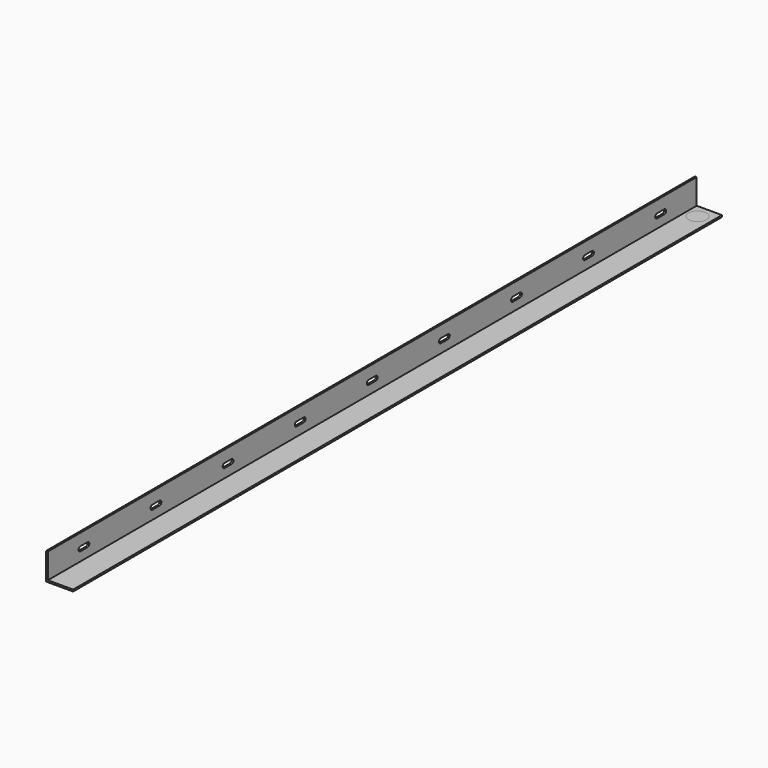
from build123d import *

# Parameters (mm, degrees)
F1_DEPTH = 400
F3_DEPTH = 2
F4_DEPTH = 900
F5_DEPTH = 2
F6_R     = 10
F7_DEPTH = 2


with BuildPart() as f1:
    # F0 (on Front) → F1 (new body)
    with BuildSketch(Plane.XZ):
        Polygon((-6.9707836596, 25.3386970109), (-8.9707836596, 25.3386970109), (-8.9707836596, -4.6613029891), (21.0292163404, -4.6613029891), (21.0292163404, -2.6613029891), (-6.9707836596, -2.6613029891), align=None)
    extrude(amount=F1_DEPTH)

    # F2 (on face) → F3 (cut)
    with BuildSketch(Plane.YZ.offset(-6.9707836596)):
        with BuildLine():
            ThreePointArc((-352.5, 9.7042359412), (-351.767766953, 11.4720028941), (-350, 12.2042359412))
            Line((-350, 12.2042359412), (-355, 12.2042359412))
            ThreePointArc((-355, 12.2042359412), (-357.5, 9.7042359412), (-355, 7.2042359412))
            Line((-355, 7.2042359412), (-350, 7.2042359412))
            ThreePointArc((-350, 7.2042359412), (-351.767766953, 7.9364689882), (-352.5, 9.7042359412))
        make_face()
        with BuildLine():
            Line((-347.5, 9.7042359412), (-350, 9.7042359412))
            Line((-350, 9.7042359412), (-350, 7.2042359412))
            ThreePointArc((-350, 7.2042359412), (-348.232233047, 7.9364689882), (-347.5, 9.7042359412))
        make_face()
        with BuildLine():
            Line((-350, 7.2042359412), (-350, 9.7042359412))
            Line((-350, 9.7042359412), (-352.5, 9.7042359412))
            ThreePointArc((-352.5, 9.7042359412), (-351.767766953, 7.9364689882), (-350, 7.2042359412))
        make_face()
        with BuildLine():
            ThreePointArc((-347.5, 9.7042359412), (-348.232233047, 11.4720028941), (-350, 12.2042359412))
            Line((-350, 12.2042359412), (-350, 9.7042359412))
            Line((-350, 9.7042359412), (-347.5, 9.7042359412))
        make_face()
        with BuildLine():
            Line((-345, 12.2042359412), (-350, 12.2042359412))
            ThreePointArc((-350, 12.2042359412), (-348.232233047, 11.4720028941), (-347.5, 9.7042359412))
            ThreePointArc((-347.5, 9.7042359412), (-348.232233047, 7.9364689882), (-350, 7.2042359412))
            Line((-350, 7.2042359412), (-345, 7.2042359412))
            ThreePointArc((-345, 7.2042359412), (-342.5, 9.7042359412), (-345, 12.2042359412))
        make_face()
        with BuildLine():
            Line((-350, 9.7042359412), (-350, 12.2042359412))
            ThreePointArc((-350, 12.2042359412), (-351.767766953, 11.4720028941), (-352.5, 9.7042359412))
            Line((-352.5, 9.7042359412), (-350, 9.7042359412))
        make_face()
        with BuildLine():
            Line((-255, 7.2042359412), (-250, 7.2042359412))
            Line((-250, 7.2042359412), (-245, 7.2042359412))
            ThreePointArc((-245, 7.2042359412), (-242.5, 9.7042359412), (-245, 12.2042359412))
            Line((-245, 12.2042359412), (-250, 12.2042359412))
            Line((-250, 12.2042359412), (-255, 12.2042359412))
            ThreePointArc((-255, 12.2042359412), (-257.5, 9.7042359412), (-255, 7.2042359412))
        make_face()
        with BuildLine():
            Line((-155, 7.2042359412), (-150, 7.2042359412))
            Line((-150, 7.2042359412), (-145, 7.2042359412))
            ThreePointArc((-145, 7.2042359412), (-142.5, 9.7042359412), (-145, 12.2042359412))
            Line((-145, 12.2042359412), (-150, 12.2042359412))
            Line((-150, 12.2042359412), (-155, 12.2042359412))
            ThreePointArc((-155, 12.2042359412), (-157.5, 9.7042359412), (-155, 7.2042359412))
        make_face()
        with BuildLine():
            Line((-55, 7.2042359412), (-50, 7.2042359412))
            Line((-50, 7.2042359412), (-45, 7.2042359412))
            ThreePointArc((-45, 7.2042359412), (-42.5, 9.7042359412), (-45, 12.2042359412))
            Line((-45, 12.2042359412), (-50, 12.2042359412))
            Line((-50, 12.2042359412), (-55, 12.2042359412))
            ThreePointArc((-55, 12.2042359412), (-57.5, 9.7042359412), (-55, 7.2042359412))
        make_face()
    extrude(amount=-F3_DEPTH, mode=Mode.SUBTRACT)


with BuildPart() as f4:
    # F0 (on Front) → F4 (new body)
    with BuildSketch(Plane.XZ):
        Polygon((-6.9707836596, 25.3386970109), (-8.9707836596, 25.3386970109), (-8.9707836596, -4.6613029891), (21.0292163404, -4.6613029891), (21.0292163404, -2.6613029891), (-6.9707836596, -2.6613029891), align=None)
    extrude(amount=F4_DEPTH)

    # F2 (on face) → F5 (cut)
    with BuildSketch(Plane.YZ.offset(-6.9707836596)):
        with BuildLine():
            ThreePointArc((-347.5, 9.7042359412), (-348.232233047, 11.4720028941), (-350, 12.2042359412))
            Line((-350, 12.2042359412), (-350, 9.7042359412))
            Line((-350, 9.7042359412), (-347.5, 9.7042359412))
        make_face()
        with BuildLine():
            Line((-345, 12.2042359412), (-350, 12.2042359412))
            ThreePointArc((-350, 12.2042359412), (-348.232233047, 11.4720028941), (-347.5, 9.7042359412))
            ThreePointArc((-347.5, 9.7042359412), (-348.232233047, 7.9364689882), (-350, 7.2042359412))
            Line((-350, 7.2042359412), (-345, 7.2042359412))
            ThreePointArc((-345, 7.2042359412), (-342.5, 9.7042359412), (-345, 12.2042359412))
        make_face()
        with BuildLine():
            ThreePointArc((-352.5, 9.7042359412), (-351.767766953, 11.4720028941), (-350, 12.2042359412))
            Line((-350, 12.2042359412), (-355, 12.2042359412))
            ThreePointArc((-355, 12.2042359412), (-357.5, 9.7042359412), (-355, 7.2042359412))
            Line((-355, 7.2042359412), (-350, 7.2042359412))
            ThreePointArc((-350, 7.2042359412), (-351.767766953, 7.9364689882), (-352.5, 9.7042359412))
        make_face()
        with BuildLine():
            Line((-350, 9.7042359412), (-350, 12.2042359412))
            ThreePointArc((-350, 12.2042359412), (-351.767766953, 11.4720028941), (-352.5, 9.7042359412))
            Line((-352.5, 9.7042359412), (-350, 9.7042359412))
        make_face()
        with BuildLine():
            Line((-347.5, 9.7042359412), (-350, 9.7042359412))
            Line((-350, 9.7042359412), (-350, 7.2042359412))
            ThreePointArc((-350, 7.2042359412), (-348.232233047, 7.9364689882), (-347.5, 9.7042359412))
        make_face()
        with BuildLine():
            Line((-350, 7.2042359412), (-350, 9.7042359412))
            Line((-350, 9.7042359412), (-352.5, 9.7042359412))
            ThreePointArc((-352.5, 9.7042359412), (-351.767766953, 7.9364689882), (-350, 7.2042359412))
        make_face()
        with BuildLine():
            Line((-255, 7.2042359412), (-250, 7.2042359412))
            Line((-250, 7.2042359412), (-245, 7.2042359412))
            ThreePointArc((-245, 7.2042359412), (-242.5, 9.7042359412), (-245, 12.2042359412))
            Line((-245, 12.2042359412), (-250, 12.2042359412))
            Line((-250, 12.2042359412), (-255, 12.2042359412))
            ThreePointArc((-255, 12.2042359412), (-257.5, 9.7042359412), (-255, 7.2042359412))
        make_face()
        with BuildLine():
            Line((-155, 7.2042359412), (-150, 7.2042359412))
            Line((-150, 7.2042359412), (-145, 7.2042359412))
            ThreePointArc((-145, 7.2042359412), (-142.5, 9.7042359412), (-145, 12.2042359412))
            Line((-145, 12.2042359412), (-150, 12.2042359412))
            Line((-150, 12.2042359412), (-155, 12.2042359412))
            ThreePointArc((-155, 12.2042359412), (-157.5, 9.7042359412), (-155, 7.2042359412))
        make_face()
        with BuildLine():
            Line((-55, 7.2042359412), (-50, 7.2042359412))
            Line((-50, 7.2042359412), (-45, 7.2042359412))
            ThreePointArc((-45, 7.2042359412), (-42.5, 9.7042359412), (-45, 12.2042359412))
            Line((-45, 12.2042359412), (-50, 12.2042359412))
            Line((-50, 12.2042359412), (-55, 12.2042359412))
            ThreePointArc((-55, 12.2042359412), (-57.5, 9.7042359412), (-55, 7.2042359412))
        make_face()
        with BuildLine():
            ThreePointArc((-445, 7.2042359412), (-442.5, 9.7042359412), (-445, 12.2042359412))
            Line((-445, 12.2042359412), (-450, 12.2042359412))
            Line((-450, 12.2042359412), (-455, 12.2042359412))
            ThreePointArc((-455, 12.2042359412), (-457.5, 9.7042359412), (-455, 7.2042359412))
            Line((-455, 7.2042359412), (-450, 7.2042359412))
            Line((-450, 7.2042359412), (-445, 7.2042359412))
        make_face()
        with BuildLine():
            ThreePointArc((-545, 7.2042359412), (-542.5, 9.7042359412), (-545, 12.2042359412))
            Line((-545, 12.2042359412), (-550, 12.2042359412))
            Line((-550, 12.2042359412), (-555, 12.2042359412))
            ThreePointArc((-555, 12.2042359412), (-557.5, 9.7042359412), (-555, 7.2042359412))
            Line((-555, 7.2042359412), (-550, 7.2042359412))
            Line((-550, 7.2042359412), (-545, 7.2042359412))
        make_face()
        with BuildLine():
            ThreePointArc((-645, 7.2042359412), (-642.5, 9.7042359412), (-645, 12.2042359412))
            Line((-645, 12.2042359412), (-650, 12.2042359412))
            Line((-650, 12.2042359412), (-655, 12.2042359412))
            ThreePointArc((-655, 12.2042359412), (-657.5, 9.7042359412), (-655, 7.2042359412))
            Line((-655, 7.2042359412), (-650, 7.2042359412))
            Line((-650, 7.2042359412), (-645, 7.2042359412))
        make_face()
        with BuildLine():
            ThreePointArc((-745, 7.2042359412), (-742.5, 9.7042359412), (-745, 12.2042359412))
            Line((-745, 12.2042359412), (-750, 12.2042359412))
            Line((-750, 12.2042359412), (-755, 12.2042359412))
            ThreePointArc((-755, 12.2042359412), (-757.5, 9.7042359412), (-755, 7.2042359412))
            Line((-755, 7.2042359412), (-750, 7.2042359412))
            Line((-750, 7.2042359412), (-745, 7.2042359412))
        make_face()
        with BuildLine():
            ThreePointArc((-845, 7.2042359412), (-842.5, 9.7042359412), (-845, 12.2042359412))
            Line((-845, 12.2042359412), (-850, 12.2042359412))
            Line((-850, 12.2042359412), (-855, 12.2042359412))
            ThreePointArc((-855, 12.2042359412), (-857.5, 9.7042359412), (-855, 7.2042359412))
            Line((-855, 7.2042359412), (-850, 7.2042359412))
            Line((-850, 7.2042359412), (-845, 7.2042359412))
        make_face()
    extrude(amount=-F5_DEPTH, mode=Mode.SUBTRACT)

    # F6 (on face) → F7 (cut)
    with BuildSketch(Plane(origin=(0, 0, -4.6613029891), x_dir=(1, 0, 0), z_dir=(0, 0, -1))):
        with Locations((6.0292163404, 15)):
            Circle(F6_R)
    extrude(amount=-F7_DEPTH, mode=Mode.SUBTRACT)


solid = Compound([f1.part, f4.part])
